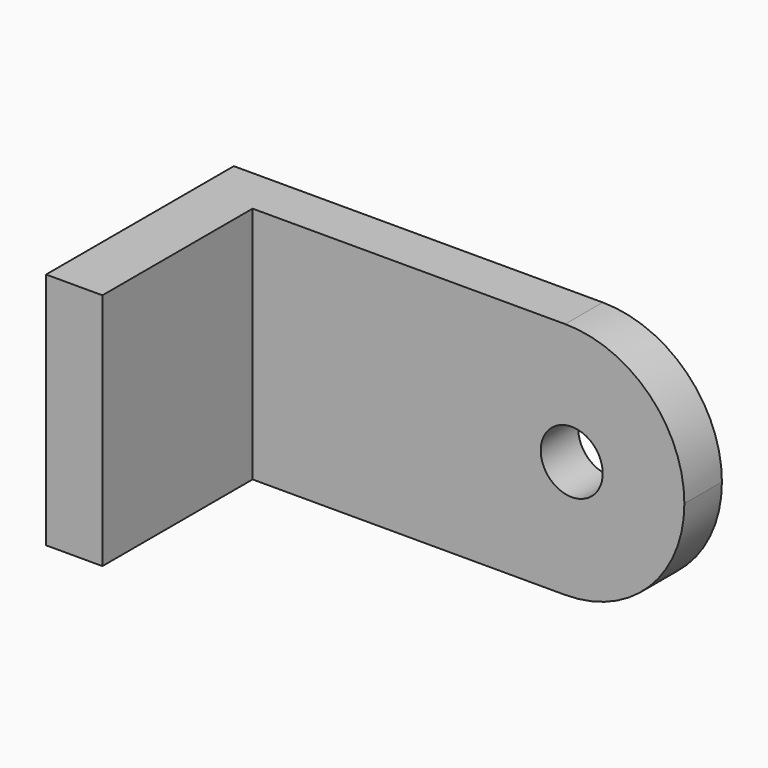
from build123d import *

# Parameters (mm, degrees)
F1_DEPTH = 12.7
F2_R     = 1.651
F3_DEPTH = 3.175
F4_R     = 6.34999


# Not quite as in the source:
# - a fillet or chamfer is up to 0.001 mm smaller than in the source, because OpenCascade refuses the exact size


with BuildPart() as f1:
    # F0 (on Top) → F1 (new body)
    with BuildSketch(Plane.XY):
        Polygon((0, -12.5), (3, -12.5), (3, -2.5), (26, -2.5), (26, 0), (0, 0), align=None)
    extrude(amount=F1_DEPTH)

    # F2 (on face) → F3 (cut)
    with BuildSketch(Plane.XZ.offset(2.5)):
        with Locations((20, 6.35)):
            Circle(F2_R)
    extrude(amount=-F3_DEPTH, mode=Mode.SUBTRACT)

    # F4 (radius 6.35 in the source; OpenCascade refuses exactly that, so slightly less here)
    f4_edges = [f1.edges().sort_by_distance(p)[0] for p in [
        (26, -1.25, 12.7),
        (26, -1.25, 0),
    ]]
    fillet(f4_edges, radius=F4_R)


solid = f1.part
